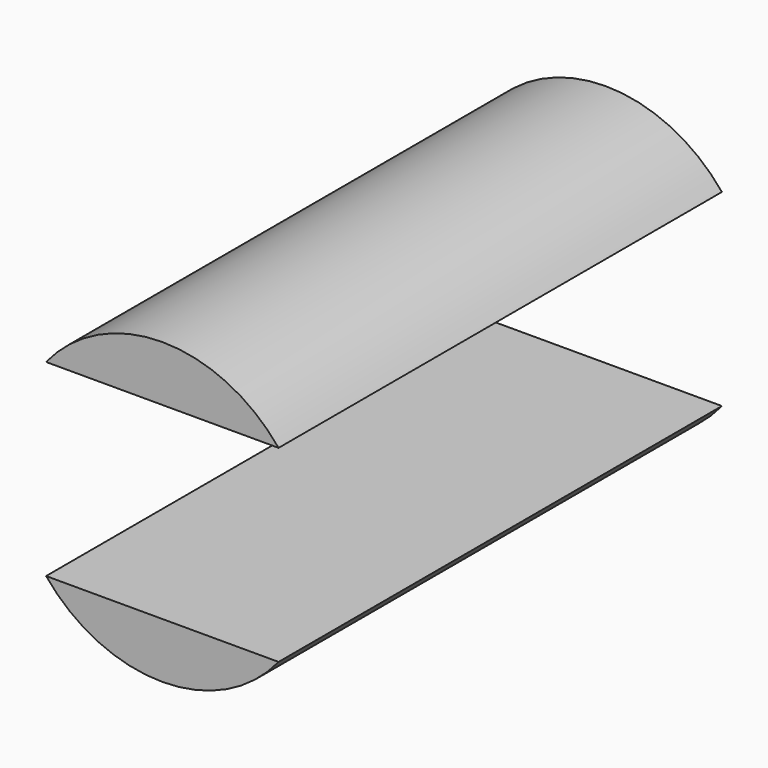
from build123d import *

# Parameters (mm, degrees)
F1_DEPTH = 6.35


# Not quite as in the source:
# - a feature names something its author has since deleted; it is built from what else it names


with BuildPart() as f1:
    # F0 (on Front) → F1 (new body)
    with BuildSketch(Plane.XZ):
        with BuildLine():
            Line((-1.3319872372, 1.0795), (1.3319872372, 1.0795))
            ThreePointArc((1.3319872372, 1.0795), (0, 1.7145), (-1.3319872372, 1.0795))
        make_face()
    extrude(amount=F1_DEPTH)


with BuildPart() as f1b:
    # F0 (on Front) → F1, piece 2 (new body)
    with BuildSketch(Plane.XZ):
        with BuildLine():
            ThreePointArc((-1.3319872372, -1.0795), (0, -1.7145), (1.3319872372, -1.0795))
            Line((1.3319872372, -1.0795), (-1.3319872372, -1.0795))
        make_face()
    extrude(amount=F1_DEPTH)


solid = Compound([f1.part, f1b.part])
